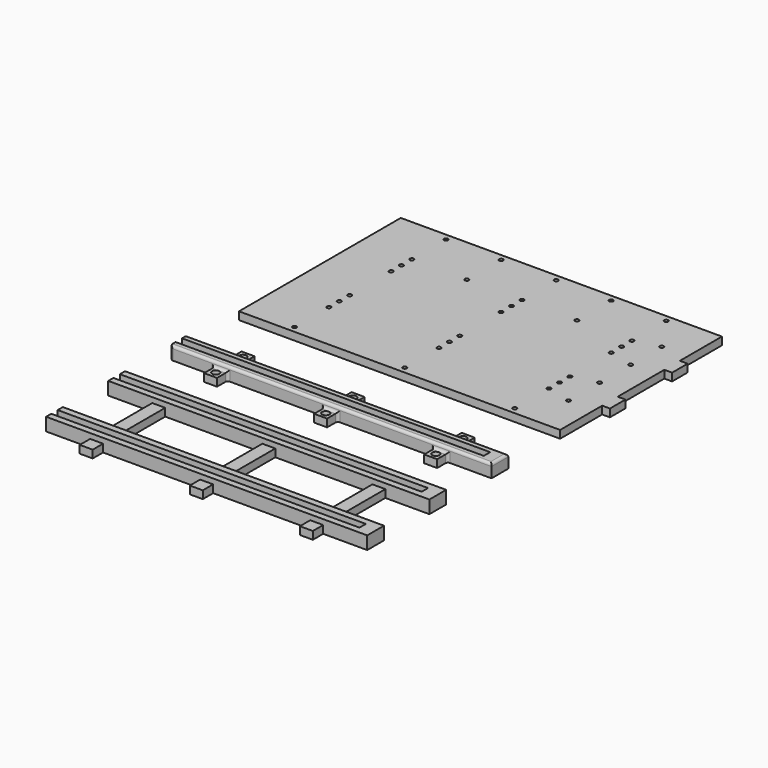
from build123d import *

# Parameters (mm, degrees)
F0_R          = 1.55
F0_W          = 6
F0_H          = 15
F1_DEPTH      = 6
F0_W_2        = 238
F0_H_2        = 6.2
F0_W_3        = 10
F2_DEPTH      = 5
F3_DEPTH      = 10
F0_H_3        = 43.8
F0_H_4        = 10
F4_DEPTH      = 6
F5_R          = 1.55
F6_DEPTH      = 20
F6_DEPTH_BACK = 25
F5_R_2        = 2.8
F7_DEPTH      = 3
F7_DEPTH_BACK = 25
F8_R          = 1.99999


# Not quite as in the source:
# - a fillet or chamfer is up to 0.001 mm smaller than in the source, because OpenCascade refuses the exact size
# - a feature names something its author has since deleted; it is built from what else it names


with BuildPart() as f1:
    # F0 (on Top) → F1 (new body)
    with BuildSketch(Plane.XY):
        Polygon((-248, 0), (0, 0), (0, 40.6), (0, 55.6), (0, 100.6), (0, 115.6), (0, 156.2), (-248, 156.2), align=None)
        with Locations((-209, 5)):
            Circle(F0_R, mode=Mode.SUBTRACT)
        with Locations((-209, 38.1)):
            Circle(F0_R, mode=Mode.SUBTRACT)
        with Locations((-209, 48.1)):
            Circle(F0_R, mode=Mode.SUBTRACT)
        with Locations((-209, 58.1)):
            Circle(F0_R, mode=Mode.SUBTRACT)
        with Locations((-209, 98.1)):
            Circle(F0_R, mode=Mode.SUBTRACT)
        with Locations((-209, 108.1)):
            Circle(F0_R, mode=Mode.SUBTRACT)
        with Locations((-209, 118.1)):
            Circle(F0_R, mode=Mode.SUBTRACT)
        with Locations((-209, 151.2)):
            Circle(F0_R, mode=Mode.SUBTRACT)
        with Locations((-124, 5)):
            Circle(F0_R, mode=Mode.SUBTRACT)
        with Locations((-124, 38.1)):
            Circle(F0_R, mode=Mode.SUBTRACT)
        with Locations((-124, 48.1)):
            Circle(F0_R, mode=Mode.SUBTRACT)
        with Locations((-124, 58.1)):
            Circle(F0_R, mode=Mode.SUBTRACT)
        with Locations((-166.5, 118.1)):
            Circle(F0_R, mode=Mode.SUBTRACT)
        with Locations((-166.5, 151.2)):
            Circle(F0_R, mode=Mode.SUBTRACT)
        with Locations((-124, 98.1)):
            Circle(F0_R, mode=Mode.SUBTRACT)
        with Locations((-124, 108.1)):
            Circle(F0_R, mode=Mode.SUBTRACT)
        with Locations((-124, 118.1)):
            Circle(F0_R, mode=Mode.SUBTRACT)
        with Locations((-124, 151.2)):
            Circle(F0_R, mode=Mode.SUBTRACT)
        with Locations((-81.5, 118.1)):
            Circle(F0_R, mode=Mode.SUBTRACT)
        with Locations((-81.5, 151.2)):
            Circle(F0_R, mode=Mode.SUBTRACT)
        with Locations((-39, 5)):
            Circle(F0_R, mode=Mode.SUBTRACT)
        with Locations((-39, 38.1)):
            Circle(F0_R, mode=Mode.SUBTRACT)
        with Locations((-39, 48.1)):
            Circle(F0_R, mode=Mode.SUBTRACT)
        with Locations((-39, 58.1)):
            Circle(F0_R, mode=Mode.SUBTRACT)
        with Locations((-20, 33.1)):
            Circle(F0_R, mode=Mode.SUBTRACT)
        with Locations((-20, 63.1)):
            Circle(F0_R, mode=Mode.SUBTRACT)
        with Locations((-39, 98.1)):
            Circle(F0_R, mode=Mode.SUBTRACT)
        with Locations((-39, 108.1)):
            Circle(F0_R, mode=Mode.SUBTRACT)
        with Locations((-39, 118.1)):
            Circle(F0_R, mode=Mode.SUBTRACT)
        with Locations((-39, 151.2)):
            Circle(F0_R, mode=Mode.SUBTRACT)
        with Locations((-20, 93.1)):
            Circle(F0_R, mode=Mode.SUBTRACT)
        with Locations((-20, 123.1)):
            Circle(F0_R, mode=Mode.SUBTRACT)
        with Locations((3, 108.1)):
            Rectangle(F0_W, F0_H)
        with Locations((3, 48.1)):
            Rectangle(F0_W, F0_H)
    extrude(amount=F1_DEPTH)


with BuildPart() as f2:
    # F0 (on Top) → F2 (new body)
    with BuildSketch(Plane.XY):
        Polygon((0, -66.2), (0, -61.2), (-10, -61.2), (-248, -61.2), (-248, -66.2), (-214, -66.2), (-204, -66.2), (-129, -66.2), (-119, -66.2), (-44, -66.2), (-34, -66.2), align=None)
        with Locations((-129, -58.1)):
            Rectangle(F0_W_2, F0_H_2)
        Polygon((0, -55), (0, -50), (-34, -50), (-44, -50), (-119, -50), (-129, -50), (-204, -50), (-214, -50), (-248, -50), (-248, -55), (-10, -55), align=None)
        with Locations((-5, -58.1)):
            Rectangle(F0_W_3, F0_H_2)
    extrude(amount=F2_DEPTH)

    # F0 (on Top) → F3, piece 2 (join)
    with BuildSketch(Plane.XY):
        Polygon((0, -66.2), (0, -61.2), (-10, -61.2), (-248, -61.2), (-248, -66.2), (-214, -66.2), (-204, -66.2), (-129, -66.2), (-119, -66.2), (-44, -66.2), (-34, -66.2), align=None)
        Polygon((0, -55), (0, -50), (-34, -50), (-44, -50), (-119, -50), (-129, -50), (-204, -50), (-214, -50), (-248, -50), (-248, -55), (-10, -55), align=None)
        with Locations((-5, -58.1)):
            Rectangle(F0_W_3, F0_H_2)
    extrude(amount=F3_DEPTH)

    # F0 (on Top) → F4, piece 2 (join)
    with BuildSketch(Plane.XY):
        with Locations((-209, -45)):
            Rectangle(F0_W_3, F0_H_4)
        with Locations((-124, -45)):
            Rectangle(F0_W_3, F0_H_4)
        with Locations((-39, -45)):
            Rectangle(F0_W_3, F0_H_4)
        with Locations((-39, -71.2)):
            Rectangle(F0_W_3, F0_H_4)
        with Locations((-124, -71.2)):
            Rectangle(F0_W_3, F0_H_4)
        with Locations((-209, -71.2)):
            Rectangle(F0_W_3, F0_H_4)
    extrude(amount=F4_DEPTH)

    # F5 (on face) → F6 (cut, two sides)
    with BuildSketch(Plane.XY.offset(6)) as f6_sk:
        with Locations((-209, -71.2)):
            Circle(F5_R)
        with Locations((-124, -71.2)):
            Circle(F5_R)
        with Locations((-39, -71.2)):
            Circle(F5_R)
        with Locations((-39, -131.2)):
            Circle(F5_R)
        with Locations((-124, -131.2)):
            Circle(F5_R)
        with Locations((-209, -131.2)):
            Circle(F5_R)
        with Locations((-209, -45)):
            Circle(F5_R)
        with Locations((-124, -45)):
            Circle(F5_R)
        with Locations((-39, -45)):
            Circle(F5_R)
    extrude(amount=-F6_DEPTH, mode=Mode.SUBTRACT)
    extrude(f6_sk.sketch, amount=F6_DEPTH_BACK, mode=Mode.SUBTRACT)

    # F5 (on face) → F7 (cut, two sides)
    with BuildSketch(Plane.XY.offset(6)) as f7_sk:
        with Locations((-209, -71.2)):
            Circle(F5_R_2)
        with Locations((-209, -71.2)):
            Circle(F5_R, mode=Mode.SUBTRACT)
        with Locations((-124, -71.2)):
            Circle(F5_R_2)
        with Locations((-124, -71.2)):
            Circle(F5_R, mode=Mode.SUBTRACT)
        with Locations((-39, -71.2)):
            Circle(F5_R_2)
        with Locations((-39, -71.2)):
            Circle(F5_R, mode=Mode.SUBTRACT)
        with Locations((-209, -131.2)):
            Circle(F5_R_2)
        with Locations((-209, -131.2)):
            Circle(F5_R, mode=Mode.SUBTRACT)
        with Locations((-124, -131.2)):
            Circle(F5_R_2)
        with Locations((-124, -131.2)):
            Circle(F5_R, mode=Mode.SUBTRACT)
        with Locations((-39, -131.2)):
            Circle(F5_R_2)
        with Locations((-39, -131.2)):
            Circle(F5_R, mode=Mode.SUBTRACT)
        with Locations((-209, -45)):
            Circle(F5_R_2)
        with Locations((-209, -45)):
            Circle(F5_R, mode=Mode.SUBTRACT)
        with Locations((-124, -45)):
            Circle(F5_R_2)
        with Locations((-124, -45)):
            Circle(F5_R, mode=Mode.SUBTRACT)
        with Locations((-39, -45)):
            Circle(F5_R_2)
        with Locations((-39, -45)):
            Circle(F5_R, mode=Mode.SUBTRACT)
    extrude(amount=-F7_DEPTH, mode=Mode.SUBTRACT)
    extrude(f7_sk.sketch, amount=F7_DEPTH_BACK, mode=Mode.SUBTRACT)

    # F8 (radius 2 in the source; OpenCascade refuses exactly that, so slightly less here)
    f8_edges = [f2.edges().sort_by_distance(p)[0] for p in [
        (-214, -66.2, 3),
        (-204, -66.2, 3),
        (-248, -66.2, 5),
        (-124, -66.2, 10),
        (-119, -66.2, 3),
        (-129, -66.2, 3),
        (0, -58.1, 10),
        (-124, -50, 10),
        (-39, -66.2, 6),
        (-44, -66.2, 3),
        (-34, -66.2, 3),
        (-34, -50, 3),
        (-39, -50, 6),
        (-44, -50, 3),
        (-124, -66.2, 6),
        (-209, -66.2, 6),
        (-209, -50, 6),
        (-204, -50, 3),
        (-214, -50, 3),
        (-129, -50, 3),
        (-124, -50, 6),
        (-119, -50, 3),
    ]]
    fillet(f8_edges, radius=F8_R)


with BuildPart() as f2b:
    # F0 (on Top) → F2, piece 2 (new body)
    with BuildSketch(Plane.XY):
        Polygon((0, -110), (-34, -110), (-44, -110), (-119, -110), (-129, -110), (-204, -110), (-214, -110), (-248, -110), (-248, -115), (-10, -115), (0, -115), align=None)
        with Locations((-129, -118.1)):
            Rectangle(F0_W_2, F0_H_2)
        Polygon((0, -126.2), (0, -121.2), (-10, -121.2), (-248, -121.2), (-248, -126.2), (-214, -126.2), (-204, -126.2), (-129, -126.2), (-119, -126.2), (-44, -126.2), (-34, -126.2), align=None)
        with Locations((-5, -118.1)):
            Rectangle(F0_W_3, F0_H_2)
    extrude(amount=F2_DEPTH)

    # F0 (on Top) → F3 (join)
    with BuildSketch(Plane.XY):
        with Locations((-5, -118.1)):
            Rectangle(F0_W_3, F0_H_2)
        Polygon((0, -110), (-34, -110), (-44, -110), (-119, -110), (-129, -110), (-204, -110), (-214, -110), (-248, -110), (-248, -115), (-10, -115), (0, -115), align=None)
        Polygon((0, -126.2), (0, -121.2), (-10, -121.2), (-248, -121.2), (-248, -126.2), (-214, -126.2), (-204, -126.2), (-129, -126.2), (-119, -126.2), (-44, -126.2), (-34, -126.2), align=None)
    extrude(amount=F3_DEPTH)



with BuildPart() as f2c:
    # F0 (on Top) → F2, piece 3 (new body)
    with BuildSketch(Plane.XY):
        Polygon((0, -170), (-34, -170), (-44, -170), (-119, -170), (-129, -170), (-204, -170), (-214, -170), (-248, -170), (-248, -175), (-10, -175), (0, -175), align=None)
        with Locations((-129, -178.1)):
            Rectangle(F0_W_2, F0_H_2)
        Polygon((0, -186.2), (0, -181.2), (-10, -181.2), (-248, -181.2), (-248, -186.2), (-214, -186.2), (-204, -186.2), (-129, -186.2), (-119, -186.2), (-44, -186.2), (-34, -186.2), align=None)
        with Locations((-5, -178.1)):
            Rectangle(F0_W_3, F0_H_2)
    extrude(amount=F2_DEPTH)

    # F0 (on Top) → F3, piece 3 (join)
    with BuildSketch(Plane.XY):
        Polygon((0, -170), (-34, -170), (-44, -170), (-119, -170), (-129, -170), (-204, -170), (-214, -170), (-248, -170), (-248, -175), (-10, -175), (0, -175), align=None)
        with Locations((-5, -178.1)):
            Rectangle(F0_W_3, F0_H_2)
        Polygon((0, -186.2), (0, -181.2), (-10, -181.2), (-248, -181.2), (-248, -186.2), (-214, -186.2), (-204, -186.2), (-129, -186.2), (-119, -186.2), (-44, -186.2), (-34, -186.2), align=None)
    extrude(amount=F3_DEPTH)


with BuildPart() as f2b_1:
    add(f2b.part)

    add(f2c.part)  # F4 merges F2c
    # F0 (on Top) → F4 (join)
    with BuildSketch(Plane.XY):
        with Locations((-39, -148.1)):
            Rectangle(F0_W_3, F0_H_3)
        with Locations((-124, -148.1)):
            Rectangle(F0_W_3, F0_H_3)
        with Locations((-209, -148.1)):
            Rectangle(F0_W_3, F0_H_3)
        with Locations((-209, -191.2)):
            Rectangle(F0_W_3, F0_H_4)
        with Locations((-124, -191.2)):
            Rectangle(F0_W_3, F0_H_4)
        with Locations((-39, -191.2)):
            Rectangle(F0_W_3, F0_H_4)
    extrude(amount=F4_DEPTH)


solid = Compound([f1.part, f2.part, f2b_1.part])
